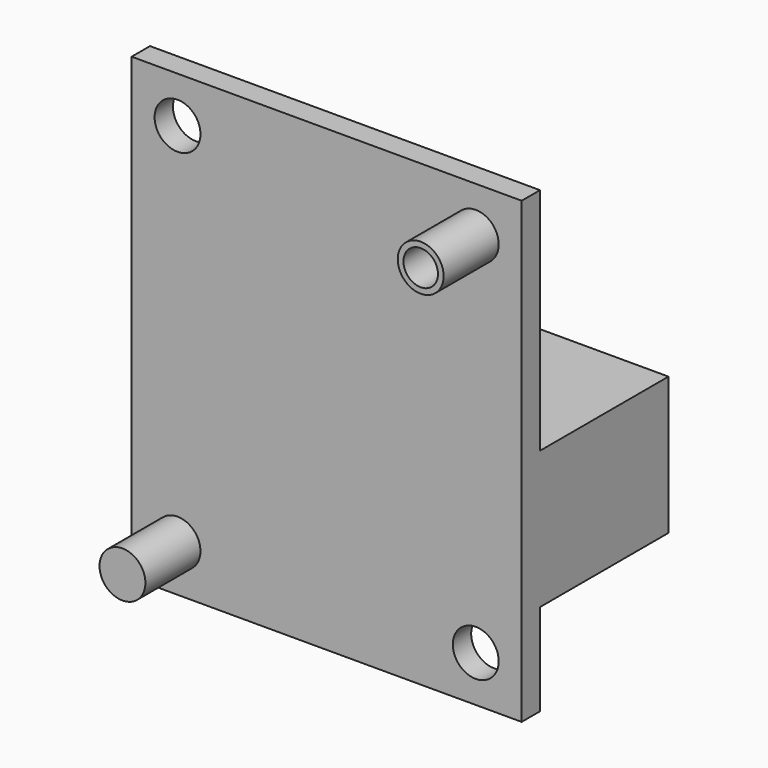
from build123d import *

# Parameters (mm, degrees)
F0_W      = 53.975
F0_H      = 12.7
F1_DEPTH  = 3.175
F3_DEPTH  = 9.525
F4_R      = 3.175
F5_DEPTH  = 3.176
F6_W      = 53.975
F6_H      = 19.05
F7_DEPTH  = 25.4
F8_W      = 53.975
F8_H      = 31.75
F9_DEPTH  = 3.175
F11_DEPTH = 25.401
F12_R     = 3.175
F13_DEPTH = 9.525
F15_DEPTH = 15.4432


# Not quite as in the source:
# - a length typed as a fraction of an inch, garbled in the dataset ("3 / 203.2 mm" for 3/8 in), is restored


with BuildPart() as f1:
    # F0 (on Front) → F1 (new body)
    with BuildSketch(Plane.XZ):
        with Locations((-7.6144175836, -40.016034618)):
            Rectangle(F0_W, F0_H)
    extrude(amount=F1_DEPTH)

    # F2 (on face) → F3 (join)
    with BuildSketch(Plane.XZ.offset(3.175)):
        with BuildLine():
            ThreePointArc((-25.0769175836, -40.016034618), (-28.2519175836, -36.841034618), (-31.4269175836, -40.016034618))
            ThreePointArc((-31.4269175836, -40.016034618), (-28.2519175836, -43.191034618), (-25.0769175836, -40.016034618))
        make_face()
    extrude(amount=F3_DEPTH)

    # F4 (on face) → F5 (cut, through all)
    with BuildSketch(Plane.XZ.offset(3.175)):
        with Locations((13.0230824164, -40.016034618)):
            Circle(F4_R)
    extrude(amount=-F5_DEPTH, mode=Mode.SUBTRACT)

    # F6 (on face) → F7 (join)
    with BuildSketch(Plane.XZ.offset(3.175)):
        with Locations((-7.6144175836, -24.141034618)):
            Rectangle(F6_W, F6_H)
    extrude(amount=-F7_DEPTH)

    # F8 (on face) → F9 (join)
    with BuildSketch(Plane.XZ.offset(3.175)):
        with Locations((-7.6144175836, 1.258965382)):
            Rectangle(F8_W, F8_H)
    extrude(amount=-F9_DEPTH)

    # F10 (on face) → F11 (cut, through all)
    with BuildSketch(Plane.XZ.offset(3.175)):
        with BuildLine():
            ThreePointArc((-25.0769175836, 10.783965382), (-28.2519175836, 13.958965382), (-31.4269175836, 10.783965382))
            ThreePointArc((-31.4269175836, 10.783965382), (-28.2519175836, 7.608965382), (-25.0769175836, 10.783965382))
        make_face()
    extrude(amount=-F11_DEPTH, mode=Mode.SUBTRACT)

    # F12 (on face) → F13 (join)
    with BuildSketch(Plane.XZ.offset(3.175)):
        with Locations((13.0230824164, 10.783965382)):
            Circle(F12_R)
    extrude(amount=F13_DEPTH)

    # F14 (on face) → F15 (cut)
    with BuildSketch(Plane(origin=(0, 0, 0), x_dir=(-1, 0, 0), z_dir=(0, 1, 0))):
        with BuildLine():
            ThreePointArc((-15.4106824164, 10.783965382), (-13.0230824164, 8.396365382), (-10.6354824164, 10.783965382))
            ThreePointArc((-10.6354824164, 10.783965382), (-13.0230824164, 13.171565382), (-15.4106824164, 10.783965382))
        make_face()
    extrude(amount=-F15_DEPTH, mode=Mode.SUBTRACT)


solid = f1.part
